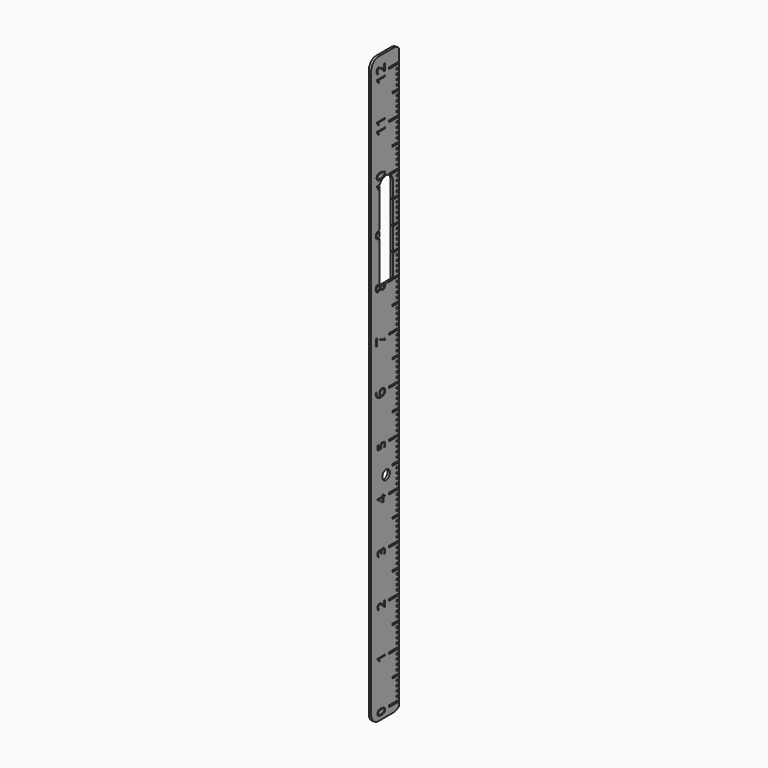
from build123d import *

# Parameters (mm, degrees)
F0_W           = 10
F0_H           = 160
F1_DEPTH       = 1
F2_W           = 4
F2_H           = 0.4
F2_W_2         = 3
F2_W_3         = 2
F2_TEXT_SIZE   = 2.7777777778
F2_TEXT_SIZE_2 = 3.4258994799
F2_TEXT_SIZE_3 = 3.0868508472
F3_DEPTH       = 5
F4_W           = 8
F4_H           = 125
F5_DEPTH       = 0.5
F6_R           = 2
F7_R           = 1
F8_DEPTH       = 12.5
F9_T1_DEPTH    = 125.3718610795
F11_W          = 25.6892092228
F11_H          = 35.3538990021
F11_W_2        = 17.939006567
F12_DEPTH      = 12.5


# Not quite as in the source:
# - a fillet or chamfer that OpenCascade refuses, or shapes differently, is made with other operations: its cross-section is extruded or revolved along the edge and cut away or added
# - Text() gives the source's letters only with a copy of the font that has no kerning and outlines rounded to 1/6400 em; it was checked with that copy


with BuildPart() as f1:
    # F0 (on Right) → F1 (new body)
    with BuildSketch(Plane.YZ):
        with Locations((-15, 80)):
            Rectangle(F0_W, F0_H)
    extrude(amount=F1_DEPTH)

    # F2 (on Right) → F3 (join, symmetric)
    with BuildSketch(Plane.YZ):
        with Locations((-12, 10.2)):
            Rectangle(F2_W, F2_H)
        with Locations((-12, 20.2)):
            Rectangle(F2_W, F2_H)
        with Locations((-12, 30.2)):
            Rectangle(F2_W, F2_H)
        with Locations((-12, 40.2)):
            Rectangle(F2_W, F2_H)
        with Locations((-12, 50.2)):
            Rectangle(F2_W, F2_H)
        with Locations((-12, 60.2)):
            Rectangle(F2_W, F2_H)
        with Locations((-12, 70.2)):
            Rectangle(F2_W, F2_H)
        with Locations((-12, 80.2)):
            Rectangle(F2_W, F2_H)
        with Locations((-12, 90.2)):
            Rectangle(F2_W, F2_H)
        with Locations((-12, 100.2)):
            Rectangle(F2_W, F2_H)
        with Locations((-12, 110.2)):
            Rectangle(F2_W, F2_H)
        with Locations((-12, 120.2)):
            Rectangle(F2_W, F2_H)
        with Locations((-12, 130.2)):
            Rectangle(F2_W, F2_H)
        with Locations((-12, 140.2)):
            Rectangle(F2_W, F2_H)
        with Locations((-11.5, 15.2)):
            Rectangle(F2_W_2, F2_H)
        with Locations((-11, 11.2)):
            Rectangle(F2_W_3, F2_H)
        with Locations((-11, 12.2)):
            Rectangle(F2_W_3, F2_H)
        with Locations((-11, 13.2)):
            Rectangle(F2_W_3, F2_H)
        with Locations((-11, 14.2)):
            Rectangle(F2_W_3, F2_H)
        with Locations((-11, 16.2)):
            Rectangle(F2_W_3, F2_H)
        with Locations((-11, 17.2)):
            Rectangle(F2_W_3, F2_H)
        with Locations((-11, 18.2)):
            Rectangle(F2_W_3, F2_H)
        with Locations((-11, 19.2)):
            Rectangle(F2_W_3, F2_H)
        with Locations((-11, 22.2)):
            Rectangle(F2_W_3, F2_H)
        with Locations((-11, 21.2)):
            Rectangle(F2_W_3, F2_H)
        with Locations((-11, 23.2)):
            Rectangle(F2_W_3, F2_H)
        with Locations((-11, 28.2)):
            Rectangle(F2_W_3, F2_H)
        with Locations((-11.5, 25.2)):
            Rectangle(F2_W_2, F2_H)
        with Locations((-11, 29.2)):
            Rectangle(F2_W_3, F2_H)
        with Locations((-11, 24.2)):
            Rectangle(F2_W_3, F2_H)
        with Locations((-11, 26.2)):
            Rectangle(F2_W_3, F2_H)
        with Locations((-11, 27.2)):
            Rectangle(F2_W_3, F2_H)
        with Locations((-11, 32.2)):
            Rectangle(F2_W_3, F2_H)
        with Locations((-11, 31.2)):
            Rectangle(F2_W_3, F2_H)
        with Locations((-11, 33.2)):
            Rectangle(F2_W_3, F2_H)
        with Locations((-11, 38.2)):
            Rectangle(F2_W_3, F2_H)
        with Locations((-11.5, 35.2)):
            Rectangle(F2_W_2, F2_H)
        with Locations((-11, 39.2)):
            Rectangle(F2_W_3, F2_H)
        with Locations((-11, 34.2)):
            Rectangle(F2_W_3, F2_H)
        with Locations((-11, 36.2)):
            Rectangle(F2_W_3, F2_H)
        with Locations((-11, 37.2)):
            Rectangle(F2_W_3, F2_H)
        with Locations((-11, 42.2)):
            Rectangle(F2_W_3, F2_H)
        with Locations((-11, 41.2)):
            Rectangle(F2_W_3, F2_H)
        with Locations((-11, 43.2)):
            Rectangle(F2_W_3, F2_H)
        with Locations((-11, 48.2)):
            Rectangle(F2_W_3, F2_H)
        with Locations((-11.5, 45.2)):
            Rectangle(F2_W_2, F2_H)
        with Locations((-11, 49.2)):
            Rectangle(F2_W_3, F2_H)
        with Locations((-11, 44.2)):
            Rectangle(F2_W_3, F2_H)
        with Locations((-11, 46.2)):
            Rectangle(F2_W_3, F2_H)
        with Locations((-11, 47.2)):
            Rectangle(F2_W_3, F2_H)
        with Locations((-11, 52.2)):
            Rectangle(F2_W_3, F2_H)
        with Locations((-11, 51.2)):
            Rectangle(F2_W_3, F2_H)
        with Locations((-11, 53.2)):
            Rectangle(F2_W_3, F2_H)
        with Locations((-11, 58.2)):
            Rectangle(F2_W_3, F2_H)
        with Locations((-11.5, 55.2)):
            Rectangle(F2_W_2, F2_H)
        with Locations((-11, 59.2)):
            Rectangle(F2_W_3, F2_H)
        with Locations((-11, 54.2)):
            Rectangle(F2_W_3, F2_H)
        with Locations((-11, 56.2)):
            Rectangle(F2_W_3, F2_H)
        with Locations((-11, 57.2)):
            Rectangle(F2_W_3, F2_H)
        with Locations((-11, 62.2)):
            Rectangle(F2_W_3, F2_H)
        with Locations((-11, 61.2)):
            Rectangle(F2_W_3, F2_H)
        with Locations((-11, 63.2)):
            Rectangle(F2_W_3, F2_H)
        with Locations((-11, 68.2)):
            Rectangle(F2_W_3, F2_H)
        with Locations((-11.5, 65.2)):
            Rectangle(F2_W_2, F2_H)
        with Locations((-11, 69.2)):
            Rectangle(F2_W_3, F2_H)
        with Locations((-11, 64.2)):
            Rectangle(F2_W_3, F2_H)
        with Locations((-11, 66.2)):
            Rectangle(F2_W_3, F2_H)
        with Locations((-11, 67.2)):
            Rectangle(F2_W_3, F2_H)
        with Locations((-11, 72.2)):
            Rectangle(F2_W_3, F2_H)
        with Locations((-11, 71.2)):
            Rectangle(F2_W_3, F2_H)
        with Locations((-11, 73.2)):
            Rectangle(F2_W_3, F2_H)
        with Locations((-11, 78.2)):
            Rectangle(F2_W_3, F2_H)
        with Locations((-11.5, 75.2)):
            Rectangle(F2_W_2, F2_H)
        with Locations((-11, 79.2)):
            Rectangle(F2_W_3, F2_H)
        with Locations((-11, 74.2)):
            Rectangle(F2_W_3, F2_H)
        with Locations((-11, 76.2)):
            Rectangle(F2_W_3, F2_H)
        with Locations((-11, 77.2)):
            Rectangle(F2_W_3, F2_H)
        with Locations((-11, 82.2)):
            Rectangle(F2_W_3, F2_H)
        with Locations((-11, 81.2)):
            Rectangle(F2_W_3, F2_H)
        with Locations((-11, 83.2)):
            Rectangle(F2_W_3, F2_H)
        with Locations((-11, 88.2)):
            Rectangle(F2_W_3, F2_H)
        with Locations((-11.5, 85.2)):
            Rectangle(F2_W_2, F2_H)
        with Locations((-11, 89.2)):
            Rectangle(F2_W_3, F2_H)
        with Locations((-11, 84.2)):
            Rectangle(F2_W_3, F2_H)
        with Locations((-11, 86.2)):
            Rectangle(F2_W_3, F2_H)
        with Locations((-11, 87.2)):
            Rectangle(F2_W_3, F2_H)
        with Locations((-11, 92.2)):
            Rectangle(F2_W_3, F2_H)
        with Locations((-11, 91.2)):
            Rectangle(F2_W_3, F2_H)
        with Locations((-11, 93.2)):
            Rectangle(F2_W_3, F2_H)
        with Locations((-11, 98.2)):
            Rectangle(F2_W_3, F2_H)
        with Locations((-11.5, 95.2)):
            Rectangle(F2_W_2, F2_H)
        with Locations((-11, 99.2)):
            Rectangle(F2_W_3, F2_H)
        with Locations((-11, 94.2)):
            Rectangle(F2_W_3, F2_H)
        with Locations((-11, 96.2)):
            Rectangle(F2_W_3, F2_H)
        with Locations((-11, 97.2)):
            Rectangle(F2_W_3, F2_H)
        with Locations((-11, 102.2)):
            Rectangle(F2_W_3, F2_H)
        with Locations((-11, 101.2)):
            Rectangle(F2_W_3, F2_H)
        with Locations((-11, 103.2)):
            Rectangle(F2_W_3, F2_H)
        with Locations((-11, 108.2)):
            Rectangle(F2_W_3, F2_H)
        with Locations((-11.5, 105.2)):
            Rectangle(F2_W_2, F2_H)
        with Locations((-11, 109.2)):
            Rectangle(F2_W_3, F2_H)
        with Locations((-11, 104.2)):
            Rectangle(F2_W_3, F2_H)
        with Locations((-11, 106.2)):
            Rectangle(F2_W_3, F2_H)
        with Locations((-11, 107.2)):
            Rectangle(F2_W_3, F2_H)
        with Locations((-11, 112.2)):
            Rectangle(F2_W_3, F2_H)
        with Locations((-11, 111.2)):
            Rectangle(F2_W_3, F2_H)
        with Locations((-11, 113.2)):
            Rectangle(F2_W_3, F2_H)
        with Locations((-11, 118.2)):
            Rectangle(F2_W_3, F2_H)
        with Locations((-11.5, 115.2)):
            Rectangle(F2_W_2, F2_H)
        with Locations((-11, 119.2)):
            Rectangle(F2_W_3, F2_H)
        with Locations((-11, 114.2)):
            Rectangle(F2_W_3, F2_H)
        with Locations((-11, 116.2)):
            Rectangle(F2_W_3, F2_H)
        with Locations((-11, 117.2)):
            Rectangle(F2_W_3, F2_H)
        with Locations((-11, 122.2)):
            Rectangle(F2_W_3, F2_H)
        with Locations((-11, 121.2)):
            Rectangle(F2_W_3, F2_H)
        with Locations((-11, 123.2)):
            Rectangle(F2_W_3, F2_H)
        with Locations((-11, 128.2)):
            Rectangle(F2_W_3, F2_H)
        with Locations((-11.5, 125.2)):
            Rectangle(F2_W_2, F2_H)
        with Locations((-11, 129.2)):
            Rectangle(F2_W_3, F2_H)
        with Locations((-11, 124.2)):
            Rectangle(F2_W_3, F2_H)
        with Locations((-11, 126.2)):
            Rectangle(F2_W_3, F2_H)
        with Locations((-11, 127.2)):
            Rectangle(F2_W_3, F2_H)
        with Locations((-11, 132.2)):
            Rectangle(F2_W_3, F2_H)
        with Locations((-11, 131.2)):
            Rectangle(F2_W_3, F2_H)
        with Locations((-11, 133.2)):
            Rectangle(F2_W_3, F2_H)
        with Locations((-11, 138.2)):
            Rectangle(F2_W_3, F2_H)
        with Locations((-11.5, 135.2)):
            Rectangle(F2_W_2, F2_H)
        with Locations((-11, 139.2)):
            Rectangle(F2_W_3, F2_H)
        with Locations((-11, 134.2)):
            Rectangle(F2_W_3, F2_H)
        with Locations((-11, 136.2)):
            Rectangle(F2_W_3, F2_H)
        with Locations((-11, 137.2)):
            Rectangle(F2_W_3, F2_H)
        with Locations(Location((-17, 10.8151041667), (0, 0, -90))):
            Text('0', F2_TEXT_SIZE, font='Open Sans', text_align=(TextAlign.LEFT, TextAlign.BOTTOM))
        with Locations(Location((-15, 19.4251302083), (0, 0, 90))):
            Text('1', F2_TEXT_SIZE, font='Open Sans', text_align=(TextAlign.LEFT, TextAlign.BOTTOM))
        with Locations(Location((-15, 29.1903211806), (0, 0, 90))):
            Text('2', F2_TEXT_SIZE, font='Open Sans', text_align=(TextAlign.LEFT, TextAlign.BOTTOM))
        with Locations(Location((-15, 39.197265625), (0, 0, 90))):
            Text('3', F2_TEXT_SIZE, font='Open Sans', text_align=(TextAlign.LEFT, TextAlign.BOTTOM))
        with Locations(Location((-15, 49.1436631944), (0, 0, 90))):
            Text('4', F2_TEXT_SIZE, font='Open Sans', text_align=(TextAlign.LEFT, TextAlign.BOTTOM))
        with Locations(Location((-15, 59.1957465278), (0, 0, 90))):
            Text('5', F2_TEXT_SIZE, font='Open Sans', text_align=(TextAlign.LEFT, TextAlign.BOTTOM))
        with Locations(Location((-15, 68.993106731), (0, 0, 90))):
            Text('6', F2_TEXT_SIZE_2, font='Open Sans', text_align=(TextAlign.LEFT, TextAlign.BOTTOM))
        with Locations(Location((-15, 78.9965861602), (0, 0, 90))):
            Text('7', F2_TEXT_SIZE_2, font='Open Sans', text_align=(TextAlign.LEFT, TextAlign.BOTTOM))
        with Locations(Location((-15, 88.9981920505), (0, 0, 90))):
            Text('8', F2_TEXT_SIZE_2, font='Open Sans', text_align=(TextAlign.LEFT, TextAlign.BOTTOM))
        with Locations(Location((-15, 99.0014038313), (0, 0, 90))):
            Text('9', F2_TEXT_SIZE_2, font='Open Sans', text_align=(TextAlign.LEFT, TextAlign.BOTTOM))
        with Locations(Location((-15, 108.2117969506), (0, 0, 90))):
            Text('10', F2_TEXT_SIZE_3, font='Open Sans', text_align=(TextAlign.LEFT, TextAlign.BOTTOM))
        with Locations(Location((-15, 118.4787613169), (0, 0, 90))):
            Text('11', F2_TEXT_SIZE_3, font='Open Sans', text_align=(TextAlign.LEFT, TextAlign.BOTTOM))
        with Locations(Location((-15, 128.2178259562), (0, 0, 90))):
            Text('12', F2_TEXT_SIZE_3, font='Open Sans', text_align=(TextAlign.LEFT, TextAlign.BOTTOM))
        with Locations(Location((-15, 138.2255430833), (0, 0, 90))):
            Text('13', F2_TEXT_SIZE_3, font='Open Sans', text_align=(TextAlign.LEFT, TextAlign.BOTTOM))
    extrude(amount=F3_DEPTH, both=True)


with BuildPart() as f5:
    # F4 (on Right) → F5 (new body)
    with BuildSketch(Plane.YZ):
        with Locations((30.2877472714, 96.0264432559)):
            Rectangle(F4_W, F4_H)
    extrude(amount=F5_DEPTH)

    # F6
    f6_edges = [f5.edges().sort_by_distance(p)[0] for p in [
        (0.25, 26.287747, 158.526443),
        (0.25, 34.287747, 158.526443),
        (0.25, 34.287747, 33.526443),
        (0.25, 26.287747, 33.526443),
    ]]
    fillet(f6_edges, radius=F6_R)

    # F7 (on face) → F8 (cut, symmetric)
    with BuildSketch(Plane.YZ.offset(0.5)):
        with BuildLine():
            Line((28.4577472714, 133.5264432559), (28.4577472714, 115.0264432559))
            Line((28.4577472714, 115.0264432559), (32.1177472714, 115.0264432559))
            Line((32.1177472714, 115.0264432559), (32.1177472714, 133.5264432559))
            ThreePointArc((32.1177472714, 133.5264432559), (30.2877472714, 135.3564432559), (28.4577472714, 133.5264432559))
        make_face()
        with Locations((30.2877472714, 79.0264432559)):
            Circle(F7_R)
    extrude(amount=F8_DEPTH, both=True, mode=Mode.SUBTRACT)

    # F9: chamfer of 0.5 on 1 edges, made by hand

    # F9_s2 → F9_t1 (cut)
    with BuildSketch(Plane.XY.offset(33.3405127162)):
        Polygon((0.5, 33.7877472714), (0, 34.2877472714), (0.5, 34.2877472714), align=None)
    extrude(amount=F9_T1_DEPTH, mode=Mode.SUBTRACT)


with BuildPart() as f1_1:
    # F10: moved
    add(f1.part.moved(Location((5.3, 45, 25))))

    # F11 (on face) → F12 (cut, symmetric)
    with BuildSketch(Plane.YZ.offset(6.3)):
        with Locations((19.1553953886, 175.4610091448)):
            Rectangle(F11_W, F11_H)
        Polygon((32, 196.6169327497), (32, 193.1379586458), (49.939006567, 193.1379586458), (49.939006567, 157.7840596437), (32, 157.7840596437), (32, 155.9), (54.170191288, 155.9), (54.170191288, 196.6169327497), align=None)
        with Locations((40.9695032835, 175.4610091448)):
            Rectangle(F11_W_2, F11_H)
    extrude(amount=F12_DEPTH, both=True, mode=Mode.SUBTRACT)


with BuildPart() as f5_1:
    add(f5.part)

    # F13: cut F1
    add(f1_1.part, mode=Mode.SUBTRACT)


solid = f5_1.part
